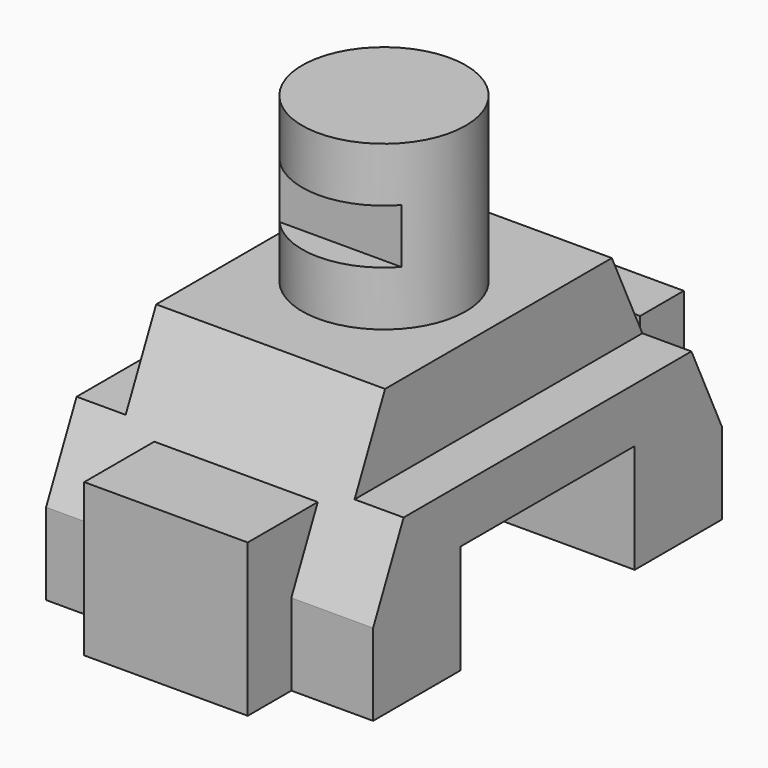
from build123d import *

# Parameters (mm, degrees)
F1_DEPTH  = 30
F2_R      = 15
F3_DEPTH  = 30
F4_W      = 30
F4_H      = 28
F5_DEPTH  = 10
F6_DEPTH  = 20
F7_W      = 9
F7_H      = 80
F8_DEPTH  = 15
F9_W      = 30
F9_H      = 10
F10_DEPTH = 40


# Not quite as in the source:
# - an extrude ends at something that could not be found from the text; its depth is read off the source's solid
# - a pattern or mirror of a feature is missing from the dataset's text; its kind, count and spacing are read off the source's solid


with BuildPart() as f1:
    # F0 (on Right) → F1 (new body, symmetric)
    with BuildSketch(Plane.YZ):
        Polygon((-20, 0), (0, 0), (20, 0), (20, -20), (40, -20), (40, -5), (26, 25), (0, 25), (-26, 25), (-40, -5), (-40, -20), (-20, -20), align=None)
    extrude(amount=F1_DEPTH, both=True)

    # F2 (on face) → F3 (join)
    with BuildSketch(Plane.XY.offset(25)):
        Circle(F2_R)
    extrude(amount=F3_DEPTH)

    # F4 (on face) → F5 (join)
    with BuildSketch(Plane.XZ.offset(40)):
        with Locations((0, -6)):
            Rectangle(F4_W, F4_H)
    f5 = extrude(amount=F5_DEPTH)

    # F5_copies: F5 across plane
    add(f5.mirror(Plane.ZX))

    # F4 (on face) → F6 (join, through all)
    with BuildSketch(Plane.XZ.offset(40)):
        with Locations((0, -6)):
            Rectangle(F4_W, F4_H)
    extrude(amount=-F6_DEPTH)

    # F7 (on face) → F8 (cut)
    with BuildSketch(Plane.XY.offset(25)):
        with Locations((25.5, 0)):
            Rectangle(F7_W, F7_H)
    f8 = extrude(amount=-F8_DEPTH, mode=Mode.SUBTRACT)

    # F8_copies: F8 across plane
    add(f8.mirror(Plane(origin=(0, 0, 0), x_dir=(0, 0, -1), z_dir=(-1, 0, 0))), mode=Mode.SUBTRACT)

    # F9 (on face) → F10 (cut)
    with BuildSketch(Plane.XZ.offset(50)):
        with Locations((0, 40)):
            Rectangle(F9_W, F9_H)
    f10 = extrude(amount=-F10_DEPTH, mode=Mode.SUBTRACT)

    # F10_copies: F10 across plane
    add(f10.mirror(Plane.ZX), mode=Mode.SUBTRACT)


solid = f1.part
